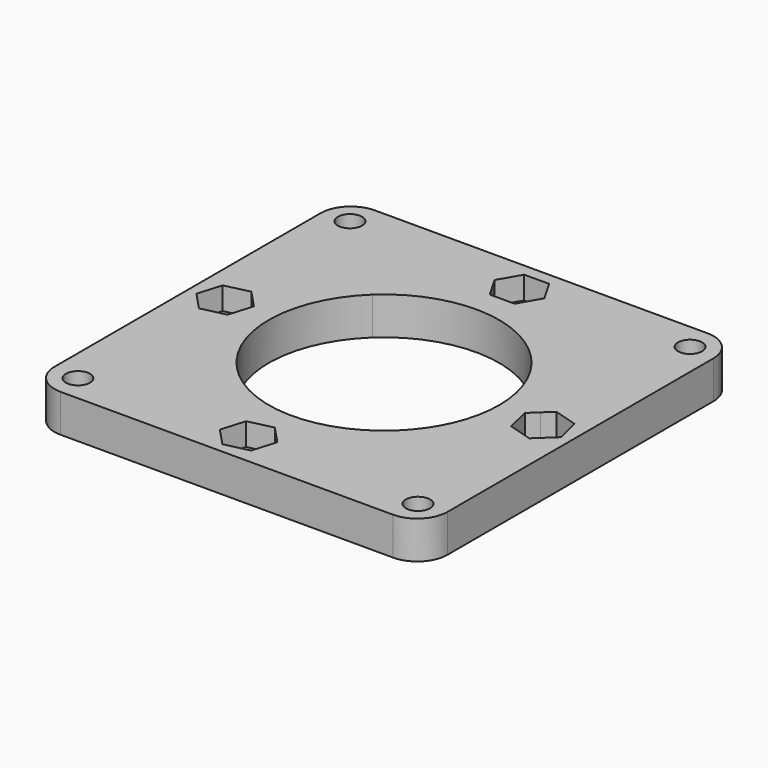
from build123d import *

# Parameters (mm, degrees)
F0_W     = 52
F0_H     = 52
F0_R     = 1.6
F1_DEPTH = 5
F2_DEPTH = 3
F3_R     = 4


# Not quite as in the source:
# - a feature names something its author has since deleted; it is built from what else it names


with BuildPart() as f1:
    # F0 (on Top) → F1 (new body)
    with BuildSketch(Plane.XY):
        Rectangle(F0_W, F0_H)
        with Locations((-22.5, -22.5)):
            Circle(F0_R, mode=Mode.SUBTRACT)
        Polygon((2.709940502, 19.3868434803), (11.1139385238, 10.4423594312), (19.6047750449, 1.4054520414), (20.8039495292, 2.5321643188), (23.9546469235, 1.5818454623), (24.7069953493, -1.6218979491), (22.3086463807, -3.875322504), (19.1579489863, -2.9250036475), (10.4423594312, -11.1139385238), (1.4054520414, -19.6047750449), (2.5321643188, -20.8039495292), (1.5818454623, -23.9546469235), (-1.6218979491, -24.7069953493), (-3.875322504, -22.3086463807), (-2.9250036475, -19.1579489863), (-11.1139385858, -10.4423593652), (-19.3028734, -1.726769876), (-22.5066168114, -2.4791183018), (-24.7600413664, -0.0807693332), (-23.8097225099, 3.0699280612), (-20.6059790985, 3.822276487), (-19.479266821, 2.6231020027), (-10.4423594312, 11.1139385238), (-1.4619546156, 19.5516867371), (-2.6193174418, 21.5562979549), (-0.9738691746, 24.4062979549), (2.3170273598, 24.4062979549), (3.962475627, 21.5562979549), align=None, mode=Mode.SUBTRACT)
        with Locations((22.5, -22.5)):
            Circle(F0_R, mode=Mode.SUBTRACT)
        with Locations((-22.5, 22.5)):
            Circle(F0_R, mode=Mode.SUBTRACT)
        with Locations((22.5, 22.5)):
            Circle(F0_R, mode=Mode.SUBTRACT)
        with BuildLine():
            ThreePointArc((-10.4423594312, 11.1139385238), (0.4748781305, 15.2426044612), (11.1139385238, 10.4423594312))
            Line((11.1139385238, 10.4423594312), (2.709940502, 19.3868434803))
            Line((2.709940502, 19.3868434803), (2.3170273598, 18.7062979549))
            Line((2.3170273598, 18.7062979549), (-0.9738691746, 18.7062979549))
            Line((-0.9738691746, 18.7062979549), (-1.4619546156, 19.5516867371))
            Line((-1.4619546156, 19.5516867371), (-10.4423594312, 11.1139385238))
        make_face()
        with BuildLine():
            ThreePointArc((11.1139385238, 10.4423594312), (14.1783296352, 5.6158230702), (15.25, 0))
            ThreePointArc((15.25, 0), (13.9965796058, -6.054606456), (10.4423594312, -11.1139385238))
            Line((10.4423594312, -11.1139385238), (19.1579489863, -2.9250036475))
            Line((19.1579489863, -2.9250036475), (18.4056005606, 0.2787397639))
            Line((18.4056005606, 0.2787397639), (19.6047750449, 1.4054520414))
            Line((19.6047750449, 1.4054520414), (11.1139385238, 10.4423594312))
        make_face()
        with BuildLine():
            Line((1.4054520414, -19.6047750449), (10.4423594312, -11.1139385238))
            ThreePointArc((10.4423594312, -11.1139385238), (-0.4748781757, -15.2426044598), (-11.1139385858, -10.4423593652))
            Line((-11.1139385858, -10.4423593652), (-2.9250036475, -19.1579489863))
            Line((-2.9250036475, -19.1579489863), (0.2787397639, -18.4056005606))
            Line((0.2787397639, -18.4056005606), (1.4054520414, -19.6047750449))
        make_face()
        with BuildLine():
            ThreePointArc((-11.1139385858, -10.4423593652), (-15.2426044598, 0.4748781757), (-10.4423594312, 11.1139385238))
            Line((-10.4423594312, 11.1139385238), (-19.479266821, 2.6231020027))
            Line((-19.479266821, 2.6231020027), (-18.3525545435, 1.4239275184))
            Line((-18.3525545435, 1.4239275184), (-19.3028734, -1.726769876))
            Line((-19.3028734, -1.726769876), (-11.1139385858, -10.4423593652))
        make_face()
        with BuildLine():
            Line((-18.3525545435, 1.4239275184), (-19.479266821, 2.6231020027))
            Line((-19.479266821, 2.6231020027), (-20.3902453885, 1.7671709018))
            ThreePointArc((-20.3902453885, 1.7671709018), (-20.0687355014, 1.2607802016), (-19.9562979549, 0.6715790926))
            ThreePointArc((-19.9562979549, 0.6715790926), (-20.087804357, 0.0363416939), (-20.4607061458, -0.4944734738))
            Line((-20.4607061458, -0.4944734738), (-19.3028734, -1.726769876))
            Line((-19.3028734, -1.726769876), (-18.3525545435, 1.4239275184))
        make_face()
        with BuildLine():
            Line((-20.3902453885, 1.7671709018), (-19.479266821, 2.6231020027))
            Line((-19.479266821, 2.6231020027), (-20.6059790985, 3.822276487))
            Line((-20.6059790985, 3.822276487), (-23.8097225099, 3.0699280612))
            Line((-23.8097225099, 3.0699280612), (-24.7600413664, -0.0807693332))
            Line((-24.7600413664, -0.0807693332), (-22.5066168114, -2.4791183018))
            Line((-22.5066168114, -2.4791183018), (-19.3028734, -1.726769876))
            Line((-19.3028734, -1.726769876), (-20.4607061458, -0.4944734738))
            ThreePointArc((-20.4607061458, -0.4944734738), (-23.1555220296, 0.7214023719), (-20.3902453885, 1.7671709018))
        make_face()
        with BuildLine():
            Line((1.7671709018, 20.3902453885), (2.709940502, 19.3868434803))
            Line((2.709940502, 19.3868434803), (3.962475627, 21.5562979549))
            Line((3.962475627, 21.5562979549), (2.3170273598, 24.4062979549))
            Line((2.3170273598, 24.4062979549), (-0.9738691746, 24.4062979549))
            Line((-0.9738691746, 24.4062979549), (-2.6193174418, 21.5562979549))
            Line((-2.6193174418, 21.5562979549), (-1.4619546156, 19.5516867371))
            Line((-1.4619546156, 19.5516867371), (-0.4944734738, 20.4607061458))
            ThreePointArc((-0.4944734738, 20.4607061458), (0.0823779836, 23.0438604085), (2.2715790926, 21.5562979549))
            ThreePointArc((2.2715790926, 21.5562979549), (2.1400726906, 20.9210605563), (1.7671709018, 20.3902453885))
        make_face()
        with BuildLine():
            Line((2.3170273598, 18.7062979549), (2.709940502, 19.3868434803))
            Line((2.709940502, 19.3868434803), (1.7671709018, 20.3902453885))
            ThreePointArc((1.7671709018, 20.3902453885), (0.6217558133, 19.9570738803), (-0.4944734738, 20.4607061458))
            Line((-0.4944734738, 20.4607061458), (-1.4619546156, 19.5516867371))
            Line((-1.4619546156, 19.5516867371), (-0.9738691746, 18.7062979549))
            Line((-0.9738691746, 18.7062979549), (2.3170273598, 18.7062979549))
        make_face()
        with BuildLine():
            Line((20.4607061458, 0.4944734738), (19.6047750449, 1.4054520414))
            Line((19.6047750449, 1.4054520414), (18.4056005606, 0.2787397639))
            Line((18.4056005606, 0.2787397639), (19.1579489863, -2.9250036475))
            Line((19.1579489863, -2.9250036475), (20.3902453885, -1.7671709018))
            ThreePointArc((20.3902453885, -1.7671709018), (19.9570738803, -0.6217558133), (20.4607061458, 0.4944734738))
        make_face()
        with BuildLine():
            Line((20.8039495292, 2.5321643188), (19.6047750449, 1.4054520414))
            Line((19.6047750449, 1.4054520414), (20.4607061458, 0.4944734738))
            ThreePointArc((20.4607061458, 0.4944734738), (22.1915353536, 0.7969145054), (23.1562979549, -0.6715790926))
            ThreePointArc((23.1562979549, -0.6715790926), (22.145499064, -2.1591415461), (20.3902453885, -1.7671709018))
            Line((20.3902453885, -1.7671709018), (19.1579489863, -2.9250036475))
            Line((19.1579489863, -2.9250036475), (22.3086463807, -3.875322504))
            Line((22.3086463807, -3.875322504), (24.7069953493, -1.6218979491))
            Line((24.7069953493, -1.6218979491), (23.9546469235, 1.5818454623))
            Line((23.9546469235, 1.5818454623), (20.8039495292, 2.5321643188))
        make_face()
        with BuildLine():
            Line((2.5321643188, -20.8039495292), (1.4054520414, -19.6047750449))
            Line((1.4054520414, -19.6047750449), (0.4944734738, -20.4607061458))
            ThreePointArc((0.4944734738, -20.4607061458), (0.8159833609, -20.9670968459), (0.9284209074, -21.5562979549))
            ThreePointArc((0.9284209074, -21.5562979549), (-1.3068164913, -23.0247915529), (-1.7671709018, -20.3902453885))
            Line((-1.7671709018, -20.3902453885), (-2.9250036475, -19.1579489863))
            Line((-2.9250036475, -19.1579489863), (-3.875322504, -22.3086463807))
            Line((-3.875322504, -22.3086463807), (-1.6218979491, -24.7069953493))
            Line((-1.6218979491, -24.7069953493), (1.5818454623, -23.9546469235))
            Line((1.5818454623, -23.9546469235), (2.5321643188, -20.8039495292))
        make_face()
        with BuildLine():
            Line((0.4944734738, -20.4607061458), (1.4054520414, -19.6047750449))
            Line((1.4054520414, -19.6047750449), (0.2787397639, -18.4056005606))
            Line((0.2787397639, -18.4056005606), (-2.9250036475, -19.1579489863))
            Line((-2.9250036475, -19.1579489863), (-1.7671709018, -20.3902453885))
            ThreePointArc((-1.7671709018, -20.3902453885), (-0.6217558133, -19.9570738803), (0.4944734738, -20.4607061458))
        make_face()
    extrude(amount=-F1_DEPTH)

    # F0 (on Top) → F2 (cut)
    with BuildSketch(Plane.XY):
        with BuildLine():
            Line((-20.3902453885, 1.7671709018), (-19.479266821, 2.6231020027))
            Line((-19.479266821, 2.6231020027), (-20.6059790985, 3.822276487))
            Line((-20.6059790985, 3.822276487), (-23.8097225099, 3.0699280612))
            Line((-23.8097225099, 3.0699280612), (-24.7600413664, -0.0807693332))
            Line((-24.7600413664, -0.0807693332), (-22.5066168114, -2.4791183018))
            Line((-22.5066168114, -2.4791183018), (-19.3028734, -1.726769876))
            Line((-19.3028734, -1.726769876), (-20.4607061458, -0.4944734738))
            ThreePointArc((-20.4607061458, -0.4944734738), (-23.1555220296, 0.7214023719), (-20.3902453885, 1.7671709018))
        make_face()
        with BuildLine():
            Line((-18.3525545435, 1.4239275184), (-19.479266821, 2.6231020027))
            Line((-19.479266821, 2.6231020027), (-20.3902453885, 1.7671709018))
            ThreePointArc((-20.3902453885, 1.7671709018), (-20.0687355014, 1.2607802016), (-19.9562979549, 0.6715790926))
            ThreePointArc((-19.9562979549, 0.6715790926), (-20.087804357, 0.0363416939), (-20.4607061458, -0.4944734738))
            Line((-20.4607061458, -0.4944734738), (-19.3028734, -1.726769876))
            Line((-19.3028734, -1.726769876), (-18.3525545435, 1.4239275184))
        make_face()
        with BuildLine():
            Line((2.3170273598, 18.7062979549), (2.709940502, 19.3868434803))
            Line((2.709940502, 19.3868434803), (1.7671709018, 20.3902453885))
            ThreePointArc((1.7671709018, 20.3902453885), (0.6217558133, 19.9570738803), (-0.4944734738, 20.4607061458))
            Line((-0.4944734738, 20.4607061458), (-1.4619546156, 19.5516867371))
            Line((-1.4619546156, 19.5516867371), (-0.9738691746, 18.7062979549))
            Line((-0.9738691746, 18.7062979549), (2.3170273598, 18.7062979549))
        make_face()
        with BuildLine():
            Line((1.7671709018, 20.3902453885), (2.709940502, 19.3868434803))
            Line((2.709940502, 19.3868434803), (3.962475627, 21.5562979549))
            Line((3.962475627, 21.5562979549), (2.3170273598, 24.4062979549))
            Line((2.3170273598, 24.4062979549), (-0.9738691746, 24.4062979549))
            Line((-0.9738691746, 24.4062979549), (-2.6193174418, 21.5562979549))
            Line((-2.6193174418, 21.5562979549), (-1.4619546156, 19.5516867371))
            Line((-1.4619546156, 19.5516867371), (-0.4944734738, 20.4607061458))
            ThreePointArc((-0.4944734738, 20.4607061458), (0.0823779836, 23.0438604085), (2.2715790926, 21.5562979549))
            ThreePointArc((2.2715790926, 21.5562979549), (2.1400726906, 20.9210605563), (1.7671709018, 20.3902453885))
        make_face()
        with BuildLine():
            Line((20.4607061458, 0.4944734738), (19.6047750449, 1.4054520414))
            Line((19.6047750449, 1.4054520414), (18.4056005606, 0.2787397639))
            Line((18.4056005606, 0.2787397639), (19.1579489863, -2.9250036475))
            Line((19.1579489863, -2.9250036475), (20.3902453885, -1.7671709018))
            ThreePointArc((20.3902453885, -1.7671709018), (19.9570738803, -0.6217558133), (20.4607061458, 0.4944734738))
        make_face()
        with BuildLine():
            Line((20.8039495292, 2.5321643188), (19.6047750449, 1.4054520414))
            Line((19.6047750449, 1.4054520414), (20.4607061458, 0.4944734738))
            ThreePointArc((20.4607061458, 0.4944734738), (22.1915353536, 0.7969145054), (23.1562979549, -0.6715790926))
            ThreePointArc((23.1562979549, -0.6715790926), (22.145499064, -2.1591415461), (20.3902453885, -1.7671709018))
            Line((20.3902453885, -1.7671709018), (19.1579489863, -2.9250036475))
            Line((19.1579489863, -2.9250036475), (22.3086463807, -3.875322504))
            Line((22.3086463807, -3.875322504), (24.7069953493, -1.6218979491))
            Line((24.7069953493, -1.6218979491), (23.9546469235, 1.5818454623))
            Line((23.9546469235, 1.5818454623), (20.8039495292, 2.5321643188))
        make_face()
        with BuildLine():
            Line((0.4944734738, -20.4607061458), (1.4054520414, -19.6047750449))
            Line((1.4054520414, -19.6047750449), (0.2787397639, -18.4056005606))
            Line((0.2787397639, -18.4056005606), (-2.9250036475, -19.1579489863))
            Line((-2.9250036475, -19.1579489863), (-1.7671709018, -20.3902453885))
            ThreePointArc((-1.7671709018, -20.3902453885), (-0.6217558133, -19.9570738803), (0.4944734738, -20.4607061458))
        make_face()
        with BuildLine():
            Line((2.5321643188, -20.8039495292), (1.4054520414, -19.6047750449))
            Line((1.4054520414, -19.6047750449), (0.4944734738, -20.4607061458))
            ThreePointArc((0.4944734738, -20.4607061458), (0.8159833609, -20.9670968459), (0.9284209074, -21.5562979549))
            ThreePointArc((0.9284209074, -21.5562979549), (-1.3068164913, -23.0247915529), (-1.7671709018, -20.3902453885))
            Line((-1.7671709018, -20.3902453885), (-2.9250036475, -19.1579489863))
            Line((-2.9250036475, -19.1579489863), (-3.875322504, -22.3086463807))
            Line((-3.875322504, -22.3086463807), (-1.6218979491, -24.7069953493))
            Line((-1.6218979491, -24.7069953493), (1.5818454623, -23.9546469235))
            Line((1.5818454623, -23.9546469235), (2.5321643188, -20.8039495292))
        make_face()
    extrude(amount=-F2_DEPTH, mode=Mode.SUBTRACT)

    # F3
    f3_edges = [f1.edges().sort_by_distance(p)[0] for p in [
        (-26, -26, -2.5),
        (26, -26, -2.5),
        (-26, 26, -2.5),
        (26, 26, -2.5),
    ]]
    fillet(f3_edges, radius=F3_R)


solid = f1.part
